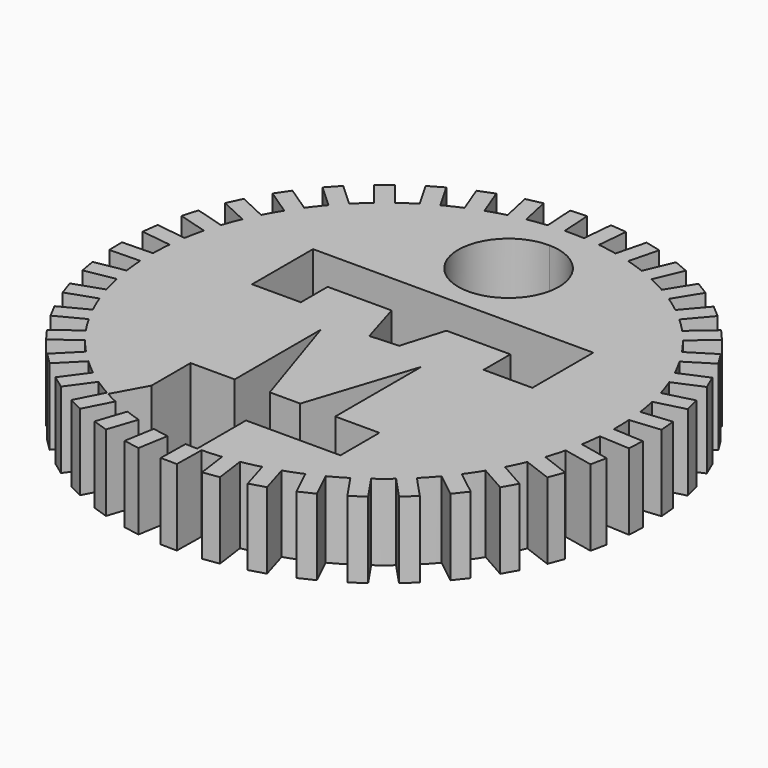
from build123d import *

# Parameters (mm, degrees)
F1_DEPTH = 25


with BuildPart() as f1:
    # F0 (on Top) → F1 (new body)
    with BuildSketch(Plane.XY):
        with BuildLine():
            Line((8.7308567075, -26.0447769336), (13.7308567075, -26.0447769336))
            Line((13.7308567075, -26.0447769336), (18.7308567075, -26.0447769336))
            Line((18.7308567075, -26.0447769336), (30.2308567075, 9.2552230664))
            Line((30.2308567075, 9.2552230664), (30.2308567075, -26.0447769336))
            Line((30.2308567075, -26.0447769336), (44.7308567075, -26.0447769336))
            Line((44.7308567075, -26.0447769336), (44.7308567075, -42.0447769336))
            Line((44.7308567075, -42.0447769336), (13.7308567075, -42.0447769336))
            Line((13.7308567075, -42.0447769336), (13.7308567075, -62.0447769336))
            ThreePointArc((13.7308567075, -62.0447769336), (14.4490545017, -62.0414111555), (15.1671892035, -62.031314117))
            ThreePointArc((15.1671892035, -62.031314117), (18.3611501979, -61.9047531443), (21.5470539818, -61.6450964616))
            ThreePointArc((21.5470539818, -61.6450964616), (24.2025899777, -61.3258794466), (26.8453677795, -60.9141800202))
            ThreePointArc((26.8453677795, -60.9141800202), (29.9825774627, -60.3015464288), (33.0915073976, -59.5586068802))
            ThreePointArc((33.0915073976, -59.5586068802), (35.6671933881, -58.8377652843), (38.2161533313, -58.0274726609))
            ThreePointArc((38.2161533313, -58.0274726609), (41.2230781673, -56.943126063), (44.1821635706, -55.7343175219))
            ThreePointArc((44.1821635706, -55.7343175219), (46.6176276591, -54.6287472612), (49.013024283, -53.4388540131))
            ThreePointArc((49.013024283, -53.4388540131), (51.8191845022, -51.9082105739), (54.55906692, -50.2618664879))
            ThreePointArc((54.55906692, -50.2618664879), (56.7972238926, -48.7974811923), (58.9829111306, -47.2558774087))
            ThreePointArc((58.9829111306, -47.2558774087), (61.5225327157, -45.3148141131), (63.9789916264, -43.2695233921))
            ThreePointArc((63.9789916264, -43.2695233921), (65.9673809805, -41.4806470118), (67.8921281763, -39.6234665789))
            ThreePointArc((67.8921281763, -39.6234665789), (70.10568455, -37.3174803054), (72.2211426387, -34.9211828304))
            ThreePointArc((72.2211426387, -34.9211828304), (73.9131582132, -32.8497451115), (75.5318509237, -30.7205187645))
            ThreePointArc((75.5318509237, -30.7205187645), (77.3674582007, -28.1036598769), (79.0923309228, -25.4125228298))
            ThreePointArc((79.0923309228, -25.4125228298), (80.4483133067, -23.1070765168), (81.7230107468, -20.7557115166))
            ThreePointArc((81.7230107468, -20.7557115166), (83.1376438483, -17.8893169692), (84.4315016491, -14.9664183215))
            ThreePointArc((84.4315016491, -14.9664183215), (85.4196677646, -12.481001122), (86.3204921067, -9.9626114713))
            ThreePointArc((86.3204921067, -9.9626114713), (87.2809932318, -6.9138671229), (88.1135091811, -3.8277171415))
            ThreePointArc((88.1135091811, -3.8277171415), (88.710697252, -1.220585128), (89.216533937, 1.4058002542))
            ThreePointArc((89.216533937, 1.4058002542), (89.7003897534, 4.5654344201), (90.0520503829, 7.7424989953))
            ThreePointArc((90.0520503829, 7.7424989953), (90.244262827, 10.410236858), (90.3432554717, 13.0830577244))
            ThreePointArc((90.3432554717, 13.0830577244), (90.3542562863, 13.8326378372), (90.3579233414, 14.5822897004))
            ThreePointArc((90.3579233414, 14.5822897004), (90.3188544192, 17.0289092933), (90.2016874917, 19.473034029))
            ThreePointArc((90.2016874917, 19.473034029), (89.9844190122, 22.1388482265), (89.674247313, 24.7954559215))
            ThreePointArc((89.674247313, 24.7954559215), (89.1822269908, 27.953829002), (88.5589131407, 31.088934161))
            ThreePointArc((88.5589131407, 31.088934161), (87.9372563266, 33.6903402679), (87.2251904452, 36.2684661586))
            ThreePointArc((87.2251904452, 36.2684661586), (86.2568130026, 39.3147178951), (85.1622325682, 42.3179325371))
            ThreePointArc((85.1622325682, 42.3179325371), (84.1507585283, 44.7939557992), (83.0534886854, 47.2331707999))
            ThreePointArc((83.0534886854, 47.2331707999), (81.631452069, 50.0958996335), (80.091261088, 52.8968309528))
            ThreePointArc((80.091261088, 52.8968309528), (78.7136779165, 55.1894354833), (77.2569231873, 57.4325664618))
            ThreePointArc((77.2569231873, 57.4325664618), (75.41455873, 60.044672455), (73.4648579735, 62.5776689954))
            ThreePointArc((73.4648579735, 62.5776689954), (71.7534550525, 64.6331180874), (69.971360533, 66.6275879546))
            ThreePointArc((69.971360533, 66.6275879546), (67.7518516962, 68.9278455569), (65.4383404976, 71.1335360264))
            ThreePointArc((65.4383404976, 71.1335360264), (63.4332316609, 72.9036516951), (61.3675681363, 74.602711768))
            ThreePointArc((61.3675681363, 74.602711768), (58.822938326, 76.5372048907), (56.1998434268, 78.3638897741))
            ThreePointArc((56.1998434268, 78.3638897741), (53.9480267261, 79.8071820086), (51.6472115988, 81.171007759))
            ThreePointArc((51.6472115988, 81.171007759), (48.8371047809, 82.6943935229), (45.9659093024, 84.0992568748))
            ThreePointArc((45.9659093024, 84.0992568748), (43.5201654127, 85.1818961284), (41.0381278389, 86.1785206366))
            ThreePointArc((41.0381278389, 86.1785206366), (38.0284105357, 87.2550921707), (34.9764128663, 88.2052051848))
            ThreePointArc((34.9764128663, 88.2052051848), (32.3940679514, 88.901815311), (29.7889847884, 89.5078785433))
            ThreePointArc((29.7889847884, 89.5078785433), (26.6502022224, 90.1124019232), (23.4889386008, 90.5854947558))
            ThreePointArc((23.4889386008, 90.5854947558), (20.8305206368, 90.8797478036), (18.1634528258, 91.0810441515))
            ThreePointArc((18.1634528258, 91.0810441515), (15.9480831486, 91.1772715715), (13.7308567075, 91.2093563344))
            ThreePointArc((13.7308567075, 91.2093563344), (12.7517199989, 91.2031003998), (11.7727431663, 91.1843336175))
            ThreePointArc((11.7727431663, 91.1843336175), (9.100563217, 91.069332545), (6.4340245672, 90.8611437927))
            ThreePointArc((6.4340245672, 90.8611437927), (3.2591234373, 90.4904588474), (0.1024442535, 89.9876854948))
            ThreePointArc((0.1024442535, 89.9876854948), (-2.5208640477, 89.4661258296), (-5.1243721306, 88.853331745))
            ThreePointArc((-5.1243721306, 88.853331745), (-8.2054799732, 88.0023446851), (-11.2484162223, 87.0235988053))
            ThreePointArc((-11.2484162223, 87.0235988053), (-13.7613647523, 86.1077054638), (-16.2408182454, 85.1046694209))
            ThreePointArc((-16.2408182454, 85.1046694209), (-19.1559142442, 83.793326662), (-22.013783712, 82.3615492287))
            ThreePointArc((-22.013783712, 82.3615492287), (-24.3574710872, 81.0727899747), (-26.6547537021, 79.7030222882))
            ThreePointArc((-26.6547537021, 79.7030222882), (-29.3355104776, 77.962060593), (-31.941327126, 76.1108112559))
            ThreePointArc((-31.941327126, 76.1108112559), (-34.0608193008, 74.4793935139), (-36.1220846801, 72.7750003774))
            ThreePointArc((-36.1220846801, 72.7750003774), (-38.5056675656, 70.6452264126), (-40.798353261, 68.4178968869))
            ThreePointArc((-40.798353261, 68.4178968869), (-42.6439711351, 66.4820597062), (-44.4209049653, 64.4829906502))
            ThreePointArc((-44.4209049653, 64.4829906502), (-46.4514447983, 62.0143245123), (-48.3772609311, 59.4631215145))
            ThreePointArc((-48.3772609311, 59.4631215145), (-49.9057447858, 57.2682392777), (-51.3566972441, 55.0213507865))
            ThreePointArc((-51.3566972441, 55.0213507865), (-52.9865998918, 52.2716559176), (-54.5004069641, 49.4563774835))
            ThreePointArc((-54.5004069641, 49.4563774835), (-55.6759304334, 47.05389637), (-56.7668924239, 44.6118536056))
            ThreePointArc((-56.7668924239, 44.6118536056), (-57.9579543497, 41.6455805227), (-59.0242700068, 38.6322143929))
            ThreePointArc((-59.0242700068, 38.6322143929), (-59.8192798169, 36.0784465237), (-60.5246801152, 33.4984888987))
            ThreePointArc((-60.5246801152, 33.4984888987), (-61.2489838371, 30.3851645288), (-61.8428145438, 27.2443414512))
            ThreePointArc((-61.8428145438, 27.2443414512), (-62.2386763385, 24.5991449807), (-62.5419809594, 21.9417445151))
            ThreePointArc((-62.5419809594, 21.9417445151), (-62.782549412, 18.7543425428), (-62.8899762798, 15.5596807483))
            Line((-62.8899762798, 15.5596807483), (-62.7715111346, 10.2125007483))
            ThreePointArc((-62.7715111346, 10.2125007483), (-62.5227055973, 7.0257311742), (-62.1412106315, 3.8521108276))
            ThreePointArc((-62.1412106315, 3.8521108276), (-61.7205135759, 1.2107503988), (-61.207890648, -1.4143188692))
            ThreePointArc((-61.207890648, -1.4143188692), (-60.4755429117, -4.5257608671), (-59.6140680309, -7.6039527947))
            ThreePointArc((-59.6140680309, -7.6039527947), (-58.7950995877, -10.1501384943), (-57.8877694384, -12.6661915398))
            ThreePointArc((-57.8877694384, -12.6661915398), (-56.6890451134, -15.6293763984), (-55.3677825587, -18.5399896972))
            ThreePointArc((-55.3677825587, -18.5399896972), (-54.169738654, -20.9313202327), (-52.8889683332, -23.279382905))
            ThreePointArc((-52.8889683332, -23.279382905), (-51.2519645016, -26.0248560826), (-49.5018835474, -28.6996684437))
            ThreePointArc((-49.5018835474, -28.6996684437), (-47.952845315, -30.8800930542), (-46.3286549934, -33.0051287543))
            ThreePointArc((-46.3286549934, -33.0051287543), (-44.2917416375, -35.4685386866), (-42.1538626981, -37.8448547754))
            ThreePointArc((-42.1538626981, -37.8448547754), (-40.2901382813, -39.7632661561), (-38.3605976033, -41.6154658483))
            ThreePointArc((-38.3605976033, -41.6154658483), (-35.9715182459, -43.7390722943), (-33.4959513917, -45.7611932758))
            ThreePointArc((-33.4959513917, -45.7611932758), (-31.3612249111, -47.3726254899), (-29.1715606749, -48.9085751833))
            ThreePointArc((-29.1715606749, -48.9085751833), (-26.4863133112, -50.6426026078), (-23.731083731, -52.2631316799))
            ThreePointArc((-23.731083731, -52.2631316799), (-23.3985286783, -52.4484202899), (-23.0650572029, -52.6320544564))
            Line((-23.0650572029, -52.6320544564), (-17.2691432925, -42.0447769336))
            Line((-17.2691432925, -42.0447769336), (-17.2691432925, -26.0447769336))
            Line((-17.2691432925, -26.0447769336), (-2.7691432925, -26.0447769336))
            Line((-2.7691432925, -26.0447769336), (-2.7691432925, 9.2552230664))
            Line((-2.7691432925, 9.2552230664), (8.7308567075, -26.0447769336))
        make_face()
        with BuildLine():
            ThreePointArc((13.7308567075, 49.4565363489), (-2.9773177291, 65.9552230664), (13.7308567075, 82.453909784))
            ThreePointArc((13.7308567075, 82.453909784), (25.2633142429, 77.5486505535), (30.0226822709, 65.9552230664))
            ThreePointArc((30.0226822709, 65.9552230664), (25.2633142429, 54.3617955793), (13.7308567075, 49.4565363489))
        make_face(mode=Mode.SUBTRACT)
        Polygon((-32.2691432925, 17.9552230664), (-32.2691432925, 42.9552230664), (13.7308567075, 42.9552230664), (59.7308567075, 42.9552230664), (59.7308567075, 17.9552230664), (43.7308567075, 17.9552230664), (43.7308567075, 28.9552230664), (22.7308567075, 28.9552230664), (18.5007124538, 14.8547422209), (13.7308567075, -1.0447769336), (9.1217184354, 14.3190173068), (4.7308567075, 28.9552230664), (-16.2691432925, 28.9552230664), (-16.2691432925, 17.9552230664), align=None, mode=Mode.SUBTRACT)
        Polygon((18.5007124538, 14.8547422209), (13.7308567075, 14.5822897004), (9.1217184354, 14.3190173068), (13.7308567075, -1.0447769336), align=None)
        with BuildLine():
            ThreePointArc((15.1671892035, -62.031314117), (14.4490545017, -62.0414111555), (13.7308567075, -62.0447769336))
            ThreePointArc((13.7308567075, -62.0447769336), (11.7744883997, -62.0197988088), (9.8193955266, -61.9448807187))
            Line((9.8193955266, -61.9448807187), (9.6577525704, -71.9460283833))
            Line((9.6577525704, -71.9460283833), (15.0055462473, -72.0324617816))
            Line((15.0055462473, -72.0324617816), (15.1671892035, -62.031314117))
        make_face()
        with BuildLine():
            ThreePointArc((-18.9769274455, -54.7135124577), (-21.0365724177, -53.7033838553), (-23.0650572029, -52.6320544564))
            ThreePointArc((-23.0650572029, -52.6320544564), (-23.3985286783, -52.4484202899), (-23.731083731, -52.2631316799))
            Line((-23.731083731, -52.2631316799), (-28.3136502011, -61.1540915607))
            Line((-28.3136502011, -61.1540915607), (-23.5594939156, -63.6044723384))
            Line((-23.5594939156, -63.6044723384), (-18.9769274455, -54.7135124577))
        make_face()
        with BuildLine():
            ThreePointArc((26.8453677795, -60.9141800202), (24.2025899777, -61.3258794466), (21.5470539818, -61.6450964616))
            Line((21.5470539818, -61.6450964616), (22.9139734449, -71.5537095954))
            Line((22.9139734449, -71.5537095954), (28.2122872426, -70.822793154))
            Line((28.2122872426, -70.822793154), (26.8453677795, -60.9141800202))
        make_face()
        with BuildLine():
            Line((-35.0576200698, -56.9958112905), (-29.1715606749, -48.9085751833))
            ThreePointArc((-29.1715606749, -48.9085751833), (-31.3612249111, -47.3726254899), (-33.4959513917, -45.7611932758))
            Line((-33.4959513917, -45.7611932758), (-39.3820107866, -53.848429383))
            Line((-39.3820107866, -53.848429383), (-35.0576200698, -56.9958112905))
        make_face()
        with BuildLine():
            ThreePointArc((38.2161533313, -58.0274726609), (35.6671933881, -58.8377652843), (33.0915073976, -59.5586068802))
            Line((33.0915073976, -59.5586068802), (35.9549498464, -69.1424359895))
            Line((35.9549498464, -69.1424359896), (41.0795957801, -67.6113017702))
            Line((41.0795957801, -67.6113017702), (38.2161533313, -58.0274726609))
        make_face()
        with BuildLine():
            Line((-45.4121856796, -48.7094202221), (-38.3605976033, -41.6154658483))
            ThreePointArc((-38.3605976033, -41.6154658483), (-40.2901382813, -39.7632661561), (-42.1538626981, -37.8448547754))
            Line((-42.1538626981, -37.8448547754), (-49.2054507744, -44.9388091491))
            Line((-49.2054507744, -44.9388091491), (-45.4121856796, -48.7094202221))
        make_face()
        with BuildLine():
            ThreePointArc((49.013024283, -53.4388540131), (46.6176276591, -54.6287472612), (44.1821635706, -55.7343175219))
            Line((44.1821635706, -55.7343175219), (48.4750123409, -64.7687257753))
            Line((48.4750123409, -64.7687257753), (53.3058730534, -62.4732622665))
            Line((53.3058730534, -62.4732622665), (49.013024283, -53.4388540131))
        make_face()
        with BuildLine():
            Line((-54.3804885031, -38.9395251167), (-46.3286549934, -33.0051287543))
            ThreePointArc((-46.3286549934, -33.0051287543), (-47.952845315, -30.8800930542), (-49.5018835474, -28.6996684437))
            Line((-49.5018835474, -28.6996684437), (-57.5537170572, -34.634064806))
            Line((-57.5537170572, -34.634064806), (-54.3804885031, -38.9395251167))
        make_face()
        with BuildLine():
            ThreePointArc((58.9829111306, -47.2558774087), (56.7972238926, -48.7974811923), (54.55906692, -50.2618664879))
            Line((54.55906692, -50.2618664879), (60.1807012752, -58.5350950131))
            Line((60.1807012752, -58.5350950131), (64.6045454857, -55.5291059339))
            Line((64.6045454857, -55.5291059339), (58.9829111306, -47.2558774087))
        make_face()
        with BuildLine():
            Line((-61.7523191234, -27.9151240349), (-52.8889683332, -23.279382905))
            ThreePointArc((-52.8889683332, -23.279382905), (-54.169738654, -20.9313202327), (-55.3677825587, -18.5399896972))
            Line((-55.3677825587, -18.5399896972), (-64.2311333489, -23.1757308271))
            Line((-64.2311333489, -23.1757308271), (-61.7523191234, -27.9151240349))
        make_face()
        with BuildLine():
            ThreePointArc((67.8921281763, -39.6234665789), (65.9673809805, -41.4806470118), (63.9789916264, -43.2695233921))
            Line((63.9789916264, -43.2695233921), (70.7976452219, -50.5876547246))
            Line((70.7976452219, -50.5876547246), (74.7107817717, -46.9415979114))
            Line((74.7107817717, -46.9415979114), (67.8921281763, -39.6234665789))
        make_face()
        with BuildLine():
            Line((-67.3548880788, -15.8946195944), (-57.8877694384, -12.6661915398))
            ThreePointArc((-57.8877694384, -12.6661915398), (-58.7950995877, -10.1501384943), (-59.6140680309, -7.6039527947))
            Line((-59.6140680309, -7.6039527947), (-69.0811866712, -10.8323808492))
            Line((-69.0811866712, -10.8323808492), (-67.3548880788, -15.8946195944))
        make_face()
        with BuildLine():
            ThreePointArc((75.5318509237, -30.7205187645), (73.9131582132, -32.8497451115), (72.2211426387, -34.9211828304))
            Line((72.2211426387, -34.9211828304), (80.0769920133, -41.1126861743))
            Line((80.0769920133, -41.1126861743), (83.3877002983, -36.9120221084))
            Line((83.3877002983, -36.9120221084), (75.5318509237, -30.7205187645))
        make_face()
        with BuildLine():
            Line((-71.0568759015, -3.159762231), (-61.207890648, -1.4143188692))
            ThreePointArc((-61.207890648, -1.4143188692), (-61.7205135759, 1.2107503988), (-62.1412106315, 3.8521108276))
            Line((-62.1412106315, 3.8521108276), (-71.990195885, 2.1066674658))
            Line((-71.990195885, 2.1066674658), (-71.0568759015, -3.159762231))
        make_face()
        with BuildLine():
            ThreePointArc((81.7230107468, -20.7557115166), (80.4483133067, -23.1070765168), (79.0923309228, -25.4125228298))
            Line((79.0923309228, -25.4125228298), (87.8012416256, -30.3322745944))
            Line((87.8012416256, -30.3322745944), (90.4319214496, -25.6754632812))
            Line((90.4319214496, -25.6754632812), (81.7230107468, -20.7557115166))
        make_face()
        with BuildLine():
            Line((-72.7715111346, 9.9909537922), (-62.7715111346, 10.2125007483))
            ThreePointArc((-62.7715111346, 10.2125007483), (-62.8774113942, 12.8850568399), (-62.8899762798, 15.5596807483))
            Line((-62.8899762798, 15.5596807483), (-72.8899762798, 15.3381337922))
            Line((-72.8899762798, 15.3381337922), (-72.7715111346, 9.9909537922))
        make_face()
        with BuildLine():
            ThreePointArc((-62.8899762798, 15.5596807483), (-62.8774113942, 12.8850568399), (-62.7715111346, 10.2125007483))
            Line((-62.7715111346, 10.2125007483), (-62.8899762798, 15.5596807483))
        make_face()
        with BuildLine():
            ThreePointArc((86.3204921067, -9.9626114713), (85.4196677646, -12.481001122), (84.4315016491, -14.9664183215))
            Line((84.4315016491, -14.9664183215), (93.7893441945, -18.4991036952))
            Line((93.7893441945, -18.4991036952), (95.6783346521, -13.495296845))
            Line((95.6783346521, -13.495296845), (86.3204921067, -9.9626114713))
        make_face()
        with BuildLine():
            Line((-72.4586041815, 23.2492868377), (-62.5419809594, 21.9417445151))
            ThreePointArc((-62.5419809594, 21.9417445151), (-62.2386763385, 24.5991449807), (-61.8428145438, 27.2443414512))
            Line((-61.8428145438, 27.2443414512), (-71.7594377658, 28.5518837737))
            Line((-71.7594377658, 28.5518837737), (-72.4586041815, 23.2492868377))
        make_face()
        with BuildLine():
            ThreePointArc((89.216533937, 1.4058002542), (88.710697252, -1.220585128), (88.1135091811, -3.8277171415))
            Line((88.1135091811, -3.8277171415), (97.9009436712, -5.8905329733))
            Line((97.9009436712, -5.8905329733), (99.0039684271, -0.6570155776))
            Line((99.0039684271, -0.6570155776), (89.216533937, 1.4058002542))
        make_face()
        with BuildLine():
            Line((-70.1254893159, 36.3044728161), (-60.5246801152, 33.4984888987))
            ThreePointArc((-60.5246801152, 33.4984888987), (-59.8192798169, 36.0784465237), (-59.0242700068, 38.6322143929))
            Line((-59.0242700068, 38.6322143929), (-68.6250792076, 41.4381983103))
            Line((-68.6250792076, 41.4381983103), (-70.1254893159, 36.3044728161))
        make_face()
        with BuildLine():
            ThreePointArc((90.3432554717, 13.0830577244), (90.244262827, 10.410236858), (90.0520503829, 7.7424989953))
            Line((90.0520503829, 7.7424989953), (100.0396676486, 7.1979033601))
            Line((100.0396676486, 7.1979033601), (100.3308727375, 12.5384620893))
            Line((100.3308727375, 12.5384620893), (90.3432554717, 13.0830577244))
        make_face()
        with BuildLine():
            Line((-65.8268527729, 48.850509233), (-56.7668924239, 44.6118536056))
            ThreePointArc((-56.7668924239, 44.6118536056), (-55.6759304334, 47.05389637), (-54.5004069641, 49.4563774835))
            Line((-54.5004069641, 49.4563774835), (-63.5603673131, 53.695033111))
            Line((-63.5603673131, 53.695033111), (-65.8268527729, 48.8505092331))
        make_face()
        with BuildLine():
            Line((-59.6634509497, 60.5933276286), (-51.3566972441, 55.0213507865))
            ThreePointArc((-51.3566972441, 55.0213507865), (-49.9057447858, 57.2682392777), (-48.3772609311, 59.4631215145))
            Line((-48.3772609311, 59.4631215145), (-56.6840146367, 65.0350983565))
            Line((-56.6840146367, 65.0350983565), (-59.6634509497, 60.5933276286))
        make_face()
        with BuildLine():
            ThreePointArc((89.674247313, 24.7954559215), (89.9844190122, 22.1388482265), (90.2016874917, 19.473034029))
            Line((90.2016874917, 19.473034029), (100.1553862496, 20.4594234506))
            Line((100.1553862496, 20.4594234506), (99.6279460709, 25.7818453431))
            Line((99.6279460709, 25.7818453431), (89.674247313, 24.7954559215))
        make_face()
        with BuildLine():
            Line((-51.7797487611, 71.2576862923), (-44.4209049653, 64.4829906502))
            ThreePointArc((-44.4209049653, 64.4829906502), (-42.6439711351, 66.4820597062), (-40.798353261, 68.4178968869))
            Line((-40.798353261, 68.4178968869), (-48.1571970567, 75.192592529))
            Line((-48.1571970567, 75.192592529), (-51.7797487611, 71.2576862923))
        make_face()
        with BuildLine():
            ThreePointArc((87.2251904452, 36.2684661586), (87.9372563266, 33.6903402679), (88.5589131407, 31.088934161))
            Line((88.5589131407, 31.088934161), (98.2453871282, 33.5831885073))
            Line((98.2453871282, 33.5831885073), (96.9116644326, 38.7627205049))
            Line((96.9116644326, 38.7627205049), (87.2251904452, 36.2684661586))
        make_face()
        with BuildLine():
            Line((-42.3605335045, 80.5936216956), (-36.1220846801, 72.7750003774))
            ThreePointArc((-36.1220846801, 72.7750003774), (-34.0608193008, 74.4793935139), (-31.941327126, 76.1108112559))
            Line((-31.941327126, 76.1108112559), (-38.1797759505, 83.9294325742))
            Line((-38.1797759505, 83.9294325742), (-42.3605335045, 80.5936216956))
        make_face()
        with BuildLine():
            ThreePointArc((83.0534886854, 47.2331707999), (84.1507585283, 44.7939557992), (85.1622325682, 42.3179325371))
            Line((85.1622325682, 42.3179325371), (94.3544390449, 46.2615886003))
            Line((94.3544390449, 46.2615886003), (92.2456951621, 51.176826863))
            Line((92.2456951621, 51.176826863), (83.0534886854, 47.2331707999))
        make_face()
        with BuildLine():
            Line((-31.6265836023, 88.3823074257), (-26.6547537021, 79.7030222882))
            ThreePointArc((-26.6547537021, 79.7030222882), (-24.3574710872, 81.0727899747), (-22.013783712, 82.3615492287))
            Line((-22.013783712, 82.3615492287), (-26.9856136121, 91.0408343662))
            Line((-26.9856136121, 91.0408343662), (-31.6265836023, 88.3823074257))
        make_face()
        with BuildLine():
            ThreePointArc((77.2569231873, 57.4325664618), (78.7136779165, 55.1894354833), (80.091261088, 52.8968309528))
            Line((80.091261088, 52.8968309528), (88.5737425249, 58.1974527772))
            Line((88.5737425249, 58.1974527772), (85.7394046242, 62.7331882862))
            Line((85.7394046242, 62.7331882862), (77.2569231873, 57.4325664618))
        make_face()
        with BuildLine():
            Line((-19.8294937423, 94.4411832902), (-16.2408182454, 85.1046694209))
            ThreePointArc((-16.2408182454, 85.1046694209), (-13.7613647523, 86.1077054638), (-11.2484162223, 87.0235988053))
            Line((-11.2484162223, 87.0235988053), (-14.8370917192, 96.3601126746))
            Line((-14.8370917192, 96.3601126746), (-19.8294937423, 94.4411832902))
        make_face()
        with BuildLine():
            ThreePointArc((69.971360533, 66.6275879546), (71.7534550525, 64.6331180874), (73.4648579735, 62.5776689954))
            Line((73.4648579735, 62.5776689954), (81.0387921953, 69.1110144981))
            Line((81.0387921953, 69.1110144981), (77.5452947548, 73.1609334573))
            Line((77.5452947548, 73.1609334573), (69.971360533, 66.6275879546))
        make_face()
        with BuildLine():
            Line((-7.2457777123, 98.6282343743), (-5.1243721306, 88.853331745))
            ThreePointArc((-5.1243721306, 88.853331745), (-2.5208640477, 89.4661258296), (0.1024442535, 89.9876854948))
            Line((0.1024442535, 89.9876854948), (-2.0189613282, 99.7625881241))
            Line((-2.0189613282, 99.7625881241), (-7.2457777123, 98.6282343743))
        make_face()
        with BuildLine():
            ThreePointArc((61.3675681363, 74.602711768), (63.4332316609, 72.9036516951), (65.4383404976, 71.1335360264))
            Line((65.4383404976, 71.1335360264), (71.9262009055, 78.7464691261))
            Line((71.9262009055, 78.7464691261), (67.8554285442, 82.2156448677))
            Line((67.8554285442, 82.2156448677), (61.3675681363, 74.602711768))
        make_face()
        with BuildLine():
            Line((5.8296128496, 100.8453197492), (6.4340245672, 90.8611437927))
            ThreePointArc((6.4340245672, 90.8611437927), (9.100563217, 91.069332545), (11.7727431663, 91.1843336175))
            Line((11.7727431663, 91.1843336175), (11.1683314487, 101.168509574))
            Line((11.1683314487, 101.168509574), (5.8296128496, 100.8453197492))
        make_face()
        with BuildLine():
            ThreePointArc((51.6472115988, 81.171007759), (53.9480267261, 79.8071820086), (56.1998434268, 78.3638897741))
            Line((56.1998434268, 78.3638897741), (61.4495600717, 86.8779697715))
            Line((61.4495600717, 86.8779697715), (56.8969282436, 89.6850877564))
            Line((56.8969282436, 89.6850877564), (51.6472115988, 81.171007759))
        make_face()
        with BuildLine():
            ThreePointArc((41.0381278389, 86.1785206366), (43.5201654127, 85.1818961284), (45.9659093024, 84.0992568748))
            Line((45.9659093024, 84.0992568748), (49.8544332755, 93.3149209509))
            Line((49.8544332755, 93.3149209509), (44.9266518121, 95.3941847128))
            Line((44.9266518121, 95.3941847128), (41.0381278389, 86.1785206366))
        make_face()
        with BuildLine():
            Line((19.0902018707, 101.0404728129), (18.1634528258, 91.0810441515))
            ThreePointArc((18.1634528258, 91.0810441515), (20.8305206368, 90.8797478036), (23.4889386008, 90.5854947558))
            Line((23.4889386008, 90.5854947558), (24.4156876457, 100.5449234172))
            Line((24.4156876457, 100.5449234172), (19.0902018707, 101.0404728129))
        make_face()
        with BuildLine():
            ThreePointArc((29.7889847884, 89.5078785433), (32.3940679514, 88.901815311), (34.9764128663, 88.2052051848))
            Line((34.9764128663, 88.2052051848), (37.4126004615, 97.9064459846))
            Line((37.4126004615, 97.9064459846), (32.2251723836, 99.2091193431))
            Line((32.2251723836, 99.2091193431), (29.7889847884, 89.5078785433))
        make_face()
    extrude(amount=-F1_DEPTH)


with BuildPart() as f1b:
    # F0 (on Top) → F1, piece 2 (new body)
    with BuildSketch(Plane.XY):
        with BuildLine():
            Line((1.7689276096, -71.2119540457), (3.4553442112, -61.352690275))
            ThreePointArc((3.4553442112, -61.352690275), (0.8115111925, -60.9478225224), (-1.8165815937, -60.4509329626))
            Line((-1.8165815937, -60.4509329626), (-3.5029981953, -70.3101967333))
            Line((-3.5029981953, -70.3101967333), (1.7689276096, -71.2119540457))
        make_face()
    extrude(amount=-F1_DEPTH)


with BuildPart() as f1c:
    # F0 (on Top) → F1, piece 3 (new body)
    with BuildSketch(Plane.XY):
        with BuildLine():
            ThreePointArc((-8.0156514773, -58.8942148619), (-10.5666971208, -58.0905127699), (-13.0881399377, -57.1982700625))
            Line((-13.0881399377, -57.1982700625), (-16.2598020089, -66.6845571528))
            Line((-16.2598020089, -66.6845571528), (-11.1873135486, -68.3805019522))
            Line((-11.1873135486, -68.3805019522), (-8.0156514773, -58.8942148619))
        make_face()
    extrude(amount=-F1_DEPTH)


solid = Compound([f1.part, f1b.part, f1c.part])
